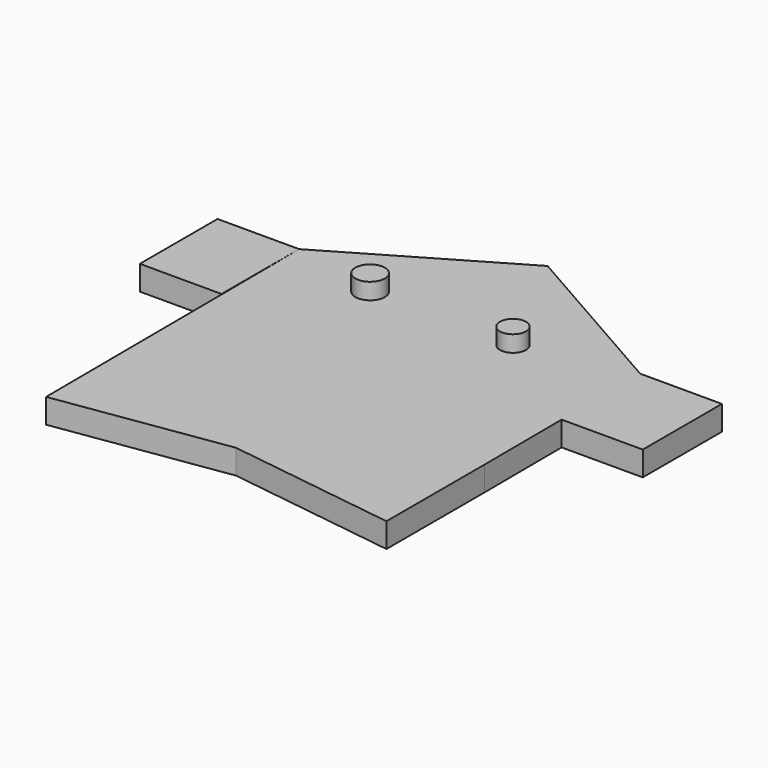
from build123d import *

# Parameters (mm, degrees)
F1_DEPTH = 7.62
F0_W     = 25.4
F0_H     = 30.1927982898
F4_R     = 4.0575582534
F5_DEPTH = 5.08
F6_R     = 4.5826589952
F7_DEPTH = 5.08


# Not quite as in the source:
# - the program builds the solid bodies; features that only make, move or delete a surface that nothing else refers to are left out


with BuildPart() as f1:
    # F0 (on Top) → F1 (new body)
    with BuildSketch(Plane.XY):
        Polygon((52.9576862357, -30.1927982898), (0.3311127876, -60.9591007506), (52.9576862357, -68.2927982898), align=None)
        Polygon((78.0265734481, 30.7663024608), (52.6265734481, 30.7663024608), (52.793687399, 0), (78.0265734481, 0), align=None)
        Polygon((0.3311127876, -60.9591007506), (-52.6265734481, -30.7663024608), (-52.4196279559, -68.86574043), align=None)
        Polygon((-0.3311127876, 60.9591007506), (-52.9576862357, 30.1927982898), (-52.6265734481, -30.7663024608), (0.3311127876, -60.9591007506), (52.9576862357, -30.1927982898), (52.793687399, 0), (52.6265734481, 0), (52.6265734481, 30.7663024608), align=None)
        Polygon((52.793687399, 0), (52.6265734481, 30.7663024608), (52.6265734481, 0), align=None)
    extrude(amount=F1_DEPTH)

    # F4 (on face) → F5 (join)
    with BuildSketch(Plane.XY.offset(7.62)):
        with Locations((19.1078484058, 23.2041683048)):
            Circle(F4_R)
    extrude(amount=F5_DEPTH)

    # F6 (on face) → F7 (join)
    with BuildSketch(Plane.XY.offset(7.62)):
        with Locations((-25.5514662713, 23.4908163548)):
            Circle(F6_R)
    extrude(amount=F7_DEPTH)


with BuildPart() as f1b:
    # F0 (on Top) → F1, piece 2 (new body)
    with BuildSketch(Plane.XY):
        with Locations((-65.6576862357, 15.0963991449)):
            Rectangle(F0_W, F0_H)
    extrude(amount=F1_DEPTH)


solid = Compound([f1.part, f1b.part])
